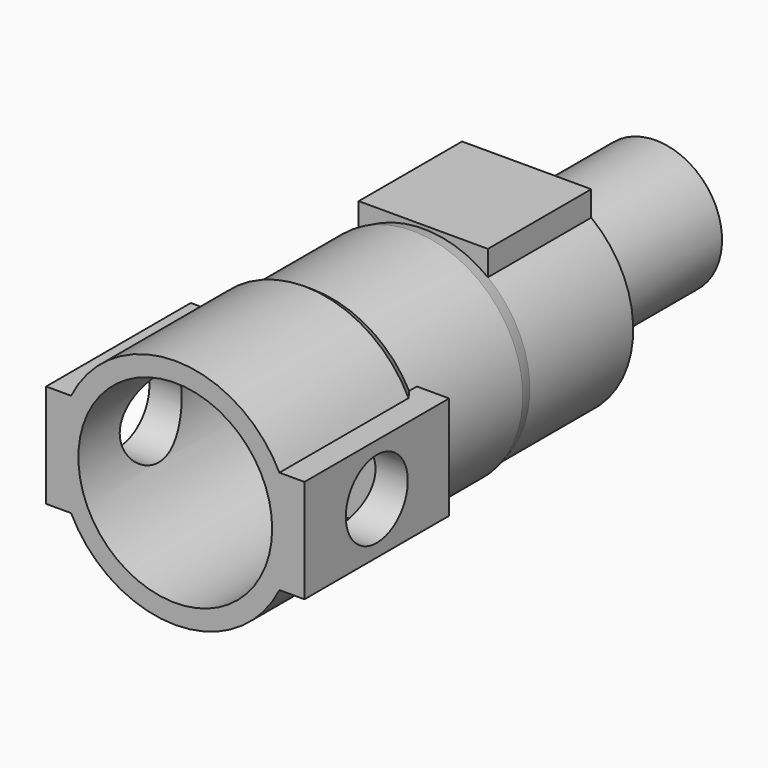
from build123d import *

# Parameters (mm, degrees)
F0_R          = 18
F0_R_2        = 15
F1_DEPTH      = 28
F3_DEPTH      = 20
F4_DEPTH      = 20
F5_R          = 9
F6_DEPTH      = 25
F7_R          = 17
F7_R_2        = 6.5
F8_DEPTH      = 20
F9_SIZE2      = 2
F9_SIZE       = 0.5
F10_DEPTH     = 20
F11_W         = 10
F11_H         = 20
F12_DEPTH     = 17
F13_R         = 15
F14_DEPTH     = 30
F15_R         = 7
F16_DEPTH     = 200
F17_T4_ANGLE  = 187.4641783336
F17_S5_R      = 17
F17_T6_DEPTH  = 27
F17_T11_ANGLE = 187.4641783336
F17_S12_R     = 17
F17_T13_DEPTH = 27
F18_R         = 10.25
F18_R_2       = 7
F19_DEPTH     = 25
F20_R         = 6
F21_DEPTH     = 45


# Not quite as in the source:
# - a fillet or chamfer that OpenCascade refuses, or shapes differently, is made with other operations: its cross-section is extruded or revolved along the edge and cut away or added


with BuildPart() as f1:
    # F0 (on Front) → F1 (new body)
    with BuildSketch(Plane.XZ):
        Circle(F0_R)
        Circle(F0_R_2, mode=Mode.SUBTRACT)
    extrude(amount=F1_DEPTH)

    # F2 (on Right) → F3 (join)
    with BuildSketch(Plane.YZ):
        Polygon((0, -8), (0, 0), (0, 8), (-28, 8), (-28, -8), align=None)
    extrude(amount=-F3_DEPTH)

    # F4 (add): a face of the model
    f4_faces = [f1.faces().sort_by_distance(p)[0] for p in [
        (0, -14, 0),
    ]]
    extrude(f4_faces, amount=F4_DEPTH)

    # F5 (on face) → F6 (cut)
    with BuildSketch(Plane.XZ.offset(28)):
        Circle(F5_R)
    extrude(amount=-F6_DEPTH, mode=Mode.SUBTRACT)

    # F7 (on face) → F8 (join)
    with BuildSketch(Plane(origin=(0, 0, 0), x_dir=(-1, 0, 0), z_dir=(0, 1, 0))):
        Circle(F7_R)
        Circle(F7_R_2, mode=Mode.SUBTRACT)
    extrude(amount=F8_DEPTH)

    # F9
    f9_edges = [f1.edges().sort_by_distance(p)[0] for p in [
        (17, 20, 0),
    ]]
    f9_side = f1.faces().sort_by_distance((16.519167, 20, 0))[0]
    chamfer(f9_edges, length=F9_SIZE, length2=F9_SIZE2, reference=f9_side)

    # F10 (add): a face of the model
    f10_faces = [f1.faces().sort_by_distance(p)[0] for p in [
        (16.0333095244, 20, 0),
    ]]
    extrude(f10_faces, amount=F10_DEPTH)

    # F11 (on Top) → F12 (join)
    with BuildSketch(Plane.XY):
        with Locations((-5, 30)):
            Rectangle(F11_W, F11_H)
        with Locations((5, 30)):
            Rectangle(F11_W, F11_H)
    extrude(amount=F12_DEPTH)

    # F13 (on face) → F14 (cut)
    with BuildSketch(Plane.XZ.offset(28)):
        Circle(F13_R)
    extrude(amount=-F14_DEPTH, mode=Mode.SUBTRACT)

    # F15 (on face) → F16 (cut)
    with BuildSketch(Plane(origin=(0, 40, 0), x_dir=(-1, 0, 0), z_dir=(0, 1, 0))):
        Circle(F15_R)
        with BuildLine():
            Line((-6.5, 0), (6.5, 0))
            ThreePointArc((6.5, 0), (0, -6.5), (-6.5, 0))
        make_face(mode=Mode.SUBTRACT)
    extrude(amount=-F16_DEPTH, mode=Mode.SUBTRACT)

    # F17: chamfer of 3 x 2 on 2 edges, made by hand


with BuildPart() as f17_tool2:
    # F17_s3 → F17_t4 (revolve)
    with BuildSketch(Plane(origin=(0, 0, 0), x_dir=(0, 1, 0), z_dir=(0.0650911923, 0, 0.9978793197))):
        with BuildLine():
            Line((0.7488452649, 15.5007698234), (-3.7488452649, 18.4992301766))
            Line((-3.7488452649, 18.4992301766), (-3.7488452649, 18.9492301766))
            ThreePointArc((-3.7488452649, 18.9492301766), (-1.8744226325, 18.45), (0, 18.45))
            Line((0, 18.45), (0.45, 18))
            ThreePointArc((0.45, 18), (0.45, 16.7503849117), (1.1988452649, 15.5007698234))
            Line((1.1988452649, 15.5007698234), (0.7488452649, 15.5007698234))
        make_face()
    revolve(axis=Axis((0, 0, 0), (0, -1, 0)), revolution_arc=F17_T4_ANGLE)

    # F17_s5 → F17_t6 (cut, symmetric)
    with BuildSketch(Plane.XZ.offset(0.9)):
        Circle(F17_S5_R)
    extrude(amount=F17_T6_DEPTH, both=True, mode=Mode.SUBTRACT)

    split(bisect_by=Plane.XY.offset(-8), keep=Keep.BOTTOM)


with BuildPart() as f1_1:
    add(f1.part)

    # F17_t1: cut F17_tool2
    add(f17_tool2.part, mode=Mode.SUBTRACT)


with BuildPart() as f17_tool9:
    # F17_s10 → F17_t11 (revolve)
    with BuildSketch(Plane(origin=(0, 0, 0), x_dir=(0, 1, 0), z_dir=(-0.0650911923, 0, -0.9978793197))):
        with BuildLine():
            Line((0.7488452649, 15.5007698234), (-3.7488452649, 18.4992301766))
            Line((-3.7488452649, 18.4992301766), (-3.7488452649, 18.9492301766))
            ThreePointArc((-3.7488452649, 18.9492301766), (-1.8744226325, 18.45), (0, 18.45))
            Line((0, 18.45), (0.45, 18))
            ThreePointArc((0.45, 18), (0.45, 16.7503849117), (1.1988452649, 15.5007698234))
            Line((1.1988452649, 15.5007698234), (0.7488452649, 15.5007698234))
        make_face()
    revolve(axis=Axis((0, 0, 0), (0, -1, 0)), revolution_arc=F17_T11_ANGLE)

    # F17_s12 → F17_t13 (cut, symmetric)
    with BuildSketch(Plane.XZ.offset(0.9)):
        Circle(F17_S12_R)
    extrude(amount=F17_T13_DEPTH, both=True, mode=Mode.SUBTRACT)

    split(bisect_by=Plane.XY.offset(8), keep=Keep.TOP)


with BuildPart() as f1_2:
    add(f1_1.part)

    # F17_t8: cut F17_tool9
    add(f17_tool9.part, mode=Mode.SUBTRACT)

    # F18 (on face) → F19 (join)
    with BuildSketch(Plane(origin=(0, 40, 0), x_dir=(-1, 0, 0), z_dir=(0, 1, 0))):
        Circle(F18_R)
        Circle(F18_R_2, mode=Mode.SUBTRACT)
    extrude(amount=F19_DEPTH)

    # F20 (on face) → F21 (cut)
    with BuildSketch(Plane(origin=(-20, 0, 0), x_dir=(0, -1, 0), z_dir=(-1, 0, 0))):
        with Locations((14, 0)):
            Circle(F20_R)
    extrude(amount=-F21_DEPTH, mode=Mode.SUBTRACT)


solid = f1_2.part
